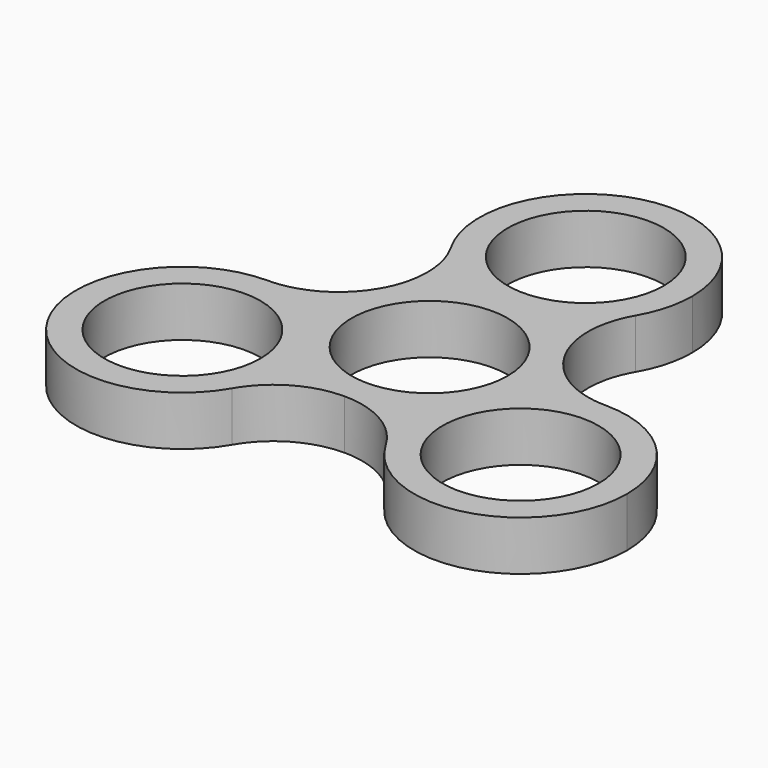
from build123d import *

# Parameters (mm, degrees)
F0_R     = 11
F1_DEPTH = 7
F2_R     = 12.499


# Not quite as in the source:
# - a fillet or chamfer is up to 0.001 mm smaller than in the source, because OpenCascade refuses the exact size


with BuildPart() as f1:
    # F0 (on Top) → F1 (new body)
    with BuildSketch(Plane.XY):
        with BuildLine():
            ThreePointArc((14.9052440041, -1.6833600857), (14.9762922658, -0.8430124372), (15, 0))
            ThreePointArc((15, 0), (12.5483433381, 8.2182163192), (5.9947894041, 13.75))
            ThreePointArc((5.9947894041, 13.75), (0, 12.5), (-5.9947894041, 13.75))
            ThreePointArc((-5.9947894041, 13.75), (-12.9903810568, 7.5), (-14.9052440041, -1.6833600857))
            ThreePointArc((-14.9052440041, -1.6833600857), (-10.8253175473, -6.25), (-8.9104546, -12.0666399143))
            ThreePointArc((-8.9104546, -12.0666399143), (0, -15), (8.9104546, -12.0666399143))
            ThreePointArc((8.9104546, -12.0666399143), (10.8253175473, -6.25), (14.9052440041, -1.6833600857))
        make_face()
        Circle(F0_R, mode=Mode.SUBTRACT)
        with BuildLine():
            ThreePointArc((-5.9947894041, 13.75), (0, 12.5), (5.9947894041, 13.75))
            ThreePointArc((5.9947894041, 13.75), (0, 15), (-5.9947894041, 13.75))
        make_face()
        with BuildLine():
            ThreePointArc((-5.9947894041, 13.75), (0, 15), (5.9947894041, 13.75))
            ThreePointArc((5.9947894041, 13.75), (12.5483433381, 19.2817836808), (15, 27.5))
            ThreePointArc((15, 27.5), (-8.2182163192, 40.0483433381), (-5.9947894041, 13.75))
        make_face()
        with Locations((0, 27.5)):
            Circle(F0_R, mode=Mode.SUBTRACT)
        with BuildLine():
            ThreePointArc((38.8156986041, -13.75), (30.5737745507, -0.3586442247), (14.9052440041, -1.6833600857))
            ThreePointArc((14.9052440041, -1.6833600857), (12.9903810568, -7.5), (8.9104546, -12.0666399143))
            ThreePointArc((8.9104546, -12.0666399143), (22.9726861669, -28.7262922658), (38.8156986041, -13.75))
        make_face()
        with Locations((23.8156986041, -13.75)):
            Circle(F0_R, mode=Mode.SUBTRACT)
        with BuildLine():
            ThreePointArc((8.9104546, -12.0666399143), (12.9903810568, -7.5), (14.9052440041, -1.6833600857))
            ThreePointArc((14.9052440041, -1.6833600857), (10.8253175473, -6.25), (8.9104546, -12.0666399143))
        make_face()
        with BuildLine():
            ThreePointArc((-8.9104546, -12.0666399143), (-10.8253175473, -6.25), (-14.9052440041, -1.6833600857))
            ThreePointArc((-14.9052440041, -1.6833600857), (-12.9903810568, -7.5), (-8.9104546, -12.0666399143))
        make_face()
        with BuildLine():
            ThreePointArc((-8.9104546, -12.0666399143), (-12.9903810568, -7.5), (-14.9052440041, -1.6833600857))
            ThreePointArc((-14.9052440041, -1.6833600857), (-37.2070543793, -20.5080759466), (-8.8156986041, -13.75))
            ThreePointArc((-8.8156986041, -13.75), (-8.8394063383, -12.9069875628), (-8.9104546, -12.0666399143))
        make_face()
        with Locations((-23.8156986041, -13.75)):
            Circle(F0_R, mode=Mode.SUBTRACT)
    extrude(amount=F1_DEPTH)

    # F2 (radius 12.5 in the source; OpenCascade refuses exactly that, so slightly less here)
    f2_edges = [f1.edges().sort_by_distance(p)[0] for p in [
        (-5.994789, 13.75, 3.5),
        (14.905244, -1.68336, 3.5),
        (-14.905244, -1.68336, 3.5),
        (5.994789, 13.75, 3.5),
        (-8.910455, -12.06664, 3.5),
        (8.910455, -12.06664, 3.5),
    ]]
    fillet(f2_edges, radius=F2_R)


solid = f1.part
